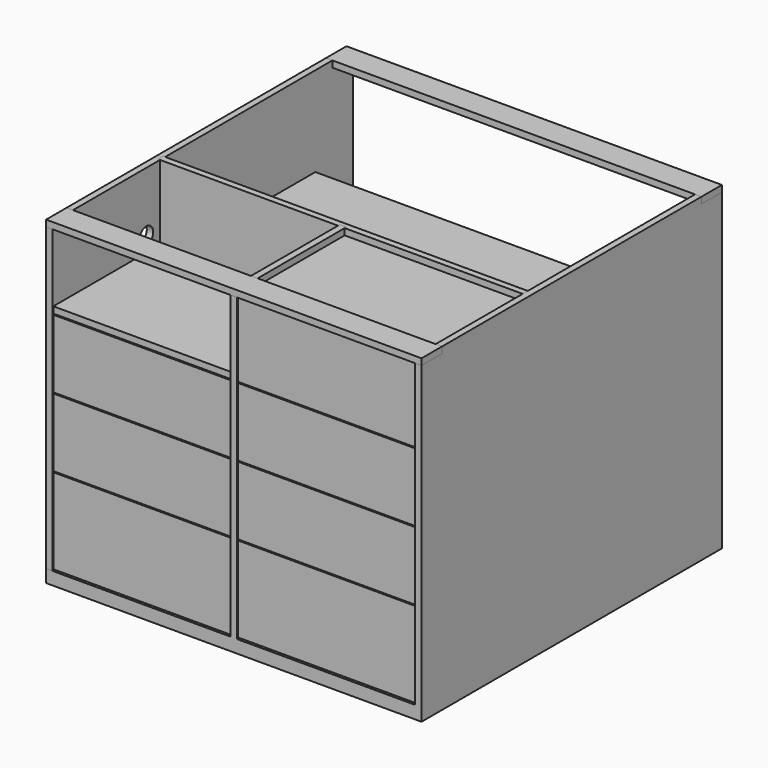
from build123d import *

# Parameters (mm, degrees)
F1_W          = 19.05
F1_H          = 914.4
F3_DEPTH      = 558.8
F3_DEPTH_BACK = 558.8
F2_W          = 19.05
F2_H          = 914.4
F4_DEPTH      = 558.8
F4_DEPTH_BACK = 558.8
F0_W          = 1117.6
F0_H          = 19.05
F5_DEPTH      = 558.8
F5_DEPTH_BACK = 558.8
F6_W          = 406.4
F6_H          = 914.4
F7_DEPTH      = 9.8425
F7_DEPTH_BACK = 9.8425
F8_W          = 76.2
F8_H          = 19.05
F9_DEPTH      = 1117.6
F11_DEPTH     = 914.4
F12_W         = 1117.6
F12_H         = 1117.6
F12_W_2       = 812.8
F12_H_2       = 812.8
F13_DEPTH     = 19.05
F14_W         = 546.1
F14_H         = 19.05
F15_DEPTH     = 396.875
F17_D         = 50.8
F17_DEPTH     = 25.4
F17_TIP       = 15.2618597233
F18_W         = 529.9075
F18_H         = 203.2
F19_DEPTH     = 396.875
F21_D         = 50.8
F21_DEPTH     = 25.4
F21_TIP       = 15.2618597233
F22_W         = 533.4
F22_H         = 203.2
F23_DEPTH     = 396.875
F24_W         = 529.9075
F24_H         = 254
F25_DEPTH     = 396.875
F24_H_2       = 203.2
F24_W_2       = 530.5425
F24_H_3       = 222.25
F26_W         = 1092.2
F26_H         = 19.05
F27_DEPTH     = 558.8


with BuildPart() as f3:
    # F1 (on Front) → F3 (new body, two sides)
    with BuildSketch(Plane.XZ) as f3_sk:
        with Locations((-549.275, 0)):
            Rectangle(F1_W, F1_H)
    extrude(amount=F3_DEPTH)
    extrude(f3_sk.sketch, amount=-F3_DEPTH_BACK)

    # F17
    with Locations(Plane.YZ.offset(-539.75)):
        with Locations((-209.55, 278.8544340611)):
            Hole(F17_D / 2, depth=F17_DEPTH)
            with Locations((0, 0, -(F17_DEPTH + F17_TIP / 2))):  # 118° drill point
                Cone(0, F17_D / 2, F17_TIP, mode=Mode.SUBTRACT)


with BuildPart() as f4:
    # F2 (on Front) → F4 (new body, two sides)
    with BuildSketch(Plane.XZ) as f4_sk:
        with Locations((549.275, 0)):
            Rectangle(F2_W, F2_H)
    extrude(amount=F4_DEPTH)
    extrude(f4_sk.sketch, amount=-F4_DEPTH_BACK)

    # F0 (on Front) → F5 (join, two sides)
    with BuildSketch(Plane.XZ) as f5_sk:
        with Locations((0, -466.725)):
            Rectangle(F0_W, F0_H)
    extrude(amount=F5_DEPTH)
    extrude(f5_sk.sketch, amount=-F5_DEPTH_BACK)

    # F6 (on Right) → F7 (join, two sides)
    with BuildSketch(Plane.YZ) as f7_sk:
        with Locations((-355.6, 0)):
            Rectangle(F6_W, F6_H)
    extrude(amount=F7_DEPTH)
    extrude(f7_sk.sketch, amount=-F7_DEPTH_BACK)

    # F12 (on face) → F13 (join)
    with BuildSketch(Plane(origin=(0, 0, -476.25), x_dir=(1, 0, 0), z_dir=(0, 0, -1))):
        Rectangle(F12_W, F12_H)
        Rectangle(F12_W_2, F12_H_2, mode=Mode.SUBTRACT)
    extrude(amount=F13_DEPTH)


with BuildPart() as f9:
    # F8 (on face) → F9 (new body)
    with BuildSketch(Plane(origin=(-558.8, 0, 0), x_dir=(0, -1, 0), z_dir=(-1, 0, 0))):
        with Locations((-520.7, 447.675)):
            Rectangle(F8_W, F8_H)
    extrude(amount=-F9_DEPTH)


with BuildPart() as f9b:
    # F8 (on face) → F9, piece 2 (new body)
    with BuildSketch(Plane(origin=(-558.8, 0, 0), x_dir=(0, -1, 0), z_dir=(-1, 0, 0))):
        with Locations((520.7, 447.675)):
            Rectangle(F8_W, F8_H)
    extrude(amount=-F9_DEPTH)


with BuildPart() as f11:
    # F10 (on face) → F11 (new body)
    with BuildSketch(Plane.XY.offset(-457.2)):
        Polygon((539.75, -139.7), (-546.1, -139.7), (-546.1, -158.75), (-9.8425, -158.75), (-9.8425, -152.4), (9.8425, -152.4), (9.8425, -158.75), (539.75, -158.75), align=None)
    extrude(amount=F11_DEPTH)

    # F21
    with Locations(Plane.XZ.offset(158.75)):
        with Locations((-60.6425, 287.2917993546)):
            Hole(F21_D / 2, depth=F21_DEPTH)
            with Locations((0, 0, -(F21_DEPTH + F21_TIP / 2))):  # 118° drill point
                Cone(0, F21_D / 2, F21_TIP, mode=Mode.SUBTRACT)


with BuildPart() as f15:
    # F14 (on face) → F15 (new body)
    with BuildSketch(Plane.XZ.offset(158.75)):
        with Locations((-275.9075, 225.425)):
            Rectangle(F14_W, F14_H)
    extrude(amount=F15_DEPTH)


with BuildPart() as f19:
    # F18 (on face) → F19 (new body)
    with BuildSketch(Plane.XZ.offset(158.75)):
        with Locations((-274.79625, 111.125)):
            Rectangle(F18_W, F18_H)
    extrude(amount=F19_DEPTH)


with BuildPart() as f23:
    # F22 (on face) → F23 (new body)
    with BuildSketch(Plane.XZ.offset(158.75)):
        with Locations((-273.05, -95.25)):
            Rectangle(F22_W, F22_H)
    extrude(amount=F23_DEPTH)


with BuildPart() as f25:
    # F24 (on face) → F25 (new body)
    with BuildSketch(Plane.XZ.offset(158.75)):
        with Locations((-274.79625, -327.025)):
            Rectangle(F24_W, F24_H)
    extrude(amount=F25_DEPTH)


with BuildPart() as f25b:
    # F24 (on face) → F25, piece 2 (new body)
    with BuildSketch(Plane.XZ.offset(158.75)):
        with Locations((274.79625, -327.025)):
            Rectangle(F24_W, F24_H)
    extrude(amount=F25_DEPTH)


with BuildPart() as f25c:
    # F24 (on face) → F25, piece 3 (new body)
    with BuildSketch(Plane.XZ.offset(158.75)):
        with Locations((274.79625, -95.25)):
            Rectangle(F24_W, F24_H_2)
    extrude(amount=F25_DEPTH)


with BuildPart() as f25d:
    # F24 (on face) → F25, piece 4 (new body)
    with BuildSketch(Plane.XZ.offset(158.75)):
        with Locations((274.47875, 111.125)):
            Rectangle(F24_W_2, F24_H_2)
    extrude(amount=F25_DEPTH)


with BuildPart() as f25e:
    # F24 (on face) → F25, piece 5 (new body)
    with BuildSketch(Plane.XZ.offset(158.75)):
        with Locations((274.79625, 327.025)):
            Rectangle(F24_W, F24_H_3)
    extrude(amount=F25_DEPTH)


with BuildPart() as f27:
    # F26 (on face) → F27 (new body)
    with BuildSketch(Plane(origin=(0, -139.7, 0), x_dir=(-1, 0, 0), z_dir=(0, 1, 0))):
        with Locations((0, 180.975)):
            Rectangle(F26_W, F26_H)
    extrude(amount=F27_DEPTH)


with BuildPart() as f27b:
    # F26 (on face) → F27, piece 2 (new body)
    with BuildSketch(Plane(origin=(0, -139.7, 0), x_dir=(-1, 0, 0), z_dir=(0, 1, 0))):
        with Locations((0, -142.875)):
            Rectangle(F26_W, F26_H)
    extrude(amount=F27_DEPTH)


solid = Compound([f3.part, f4.part, f9.part, f9b.part, f11.part, f15.part, f19.part, f23.part, f25.part, f25b.part, f25c.part, f25d.part, f25e.part, f27.part, f27b.part])
